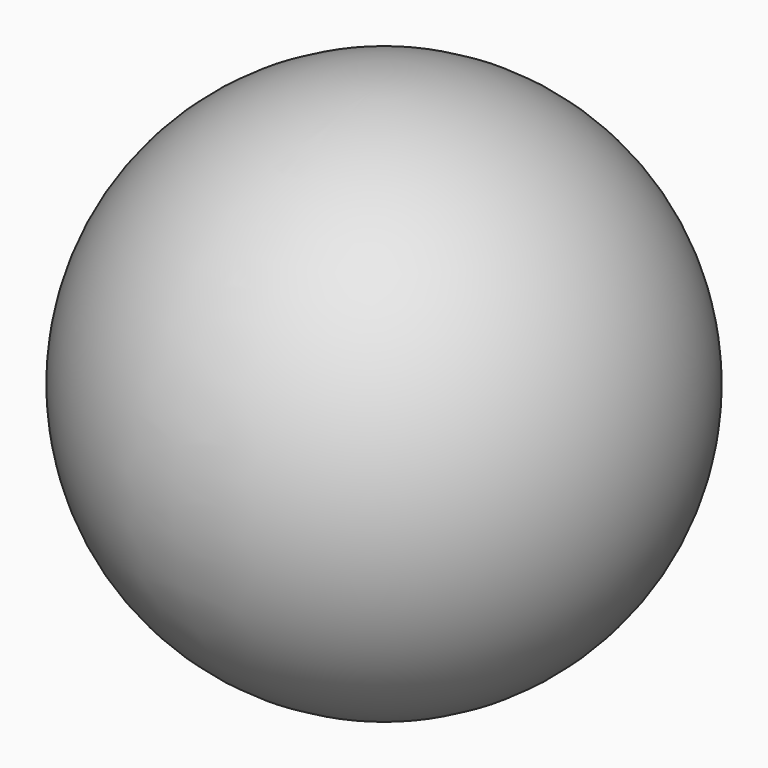
from build123d import *

# Parameters (mm, degrees)
F4_T = -2.54


# Not quite as in the source:
# - the program builds the solid bodies; features that only make, move or delete a surface that nothing else refers to are left out


with BuildPart() as f1:
    # F0 (on Right) → F1 (revolve)
    with BuildSketch(Plane.YZ):
        with BuildLine():
            Line((0, -36.8053336478), (0, 36.8053336478))
            ThreePointArc((0, 36.8053336478), (-36.8053336478, 0), (0, -36.8053336478))
        make_face()
    revolve(axis=Axis((0, 0, 0), (0, 0, -1)))

    # F4 (hollow: no face is removed)
    offset(amount=F4_T, mode=Mode.SUBTRACT)


solid = f1.part
